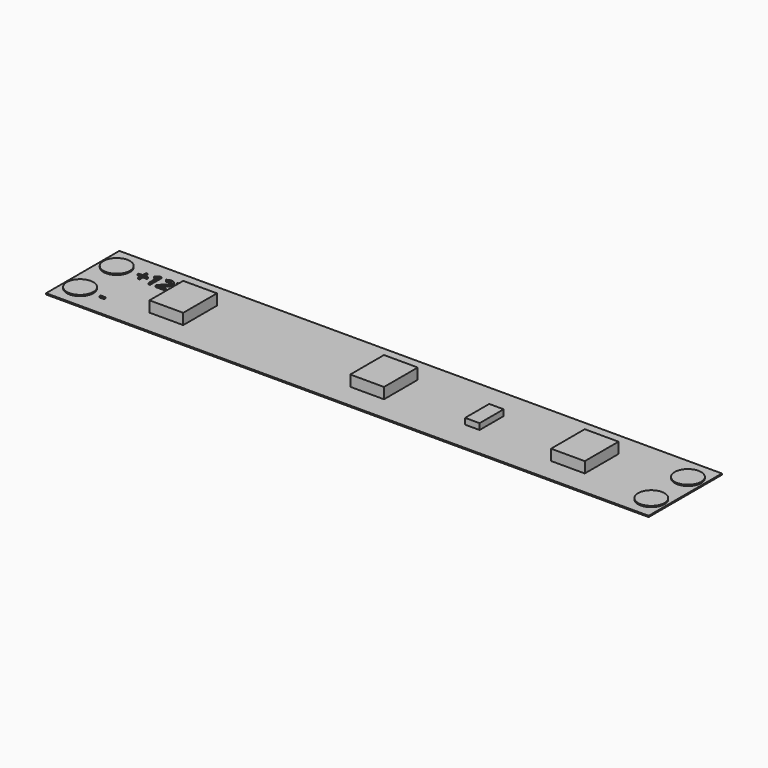
from build123d import *

# Parameters (mm, degrees)
F0_W         = 50
F0_H         = 7.6
F0_R         = 1.1
F0_W_2       = 0.3994791667
F0_H_2       = 0.1236979167
F0_W_3       = 2.8
F0_H_3       = 3.5
F0_W_4       = 1.2
F0_H_4       = 2.5
F0_TEXT_SIZE = 1.6666666667
F1_DEPTH     = 0.1
F2_DEPTH     = 0.9
F3_DEPTH     = 0.9
F4_DEPTH     = 0.5
F5_DEPTH     = 0.1
F6_DEPTH     = 0.1


# Not quite as in the source:
# - Text() gives the source's letters only with a copy of the font that has no kerning and outlines rounded to 1/6400 em; it was checked with that copy


with BuildPart() as f1:
    # F0 (on Top) → F1 (new body)
    with BuildSketch(Plane.XY):
        Rectangle(F0_W, F0_H)
        with Locations((-23.7, -1.9)):
            Circle(F0_R, mode=Mode.SUBTRACT)
        with Locations((-21.7317708333, -2.0532552083)):
            Rectangle(F0_W_2, F0_H_2, mode=Mode.SUBTRACT)
        with Locations((-16.66, 0)):
            Rectangle(F0_W_3, F0_H_3, mode=Mode.SUBTRACT)
        with Locations((23.7, -1.9)):
            Circle(F0_R, mode=Mode.SUBTRACT)
        Rectangle(F0_W_3, F0_H_3, mode=Mode.SUBTRACT)
        with Locations((8.33, 0)):
            Rectangle(F0_W_4, F0_H_4, mode=Mode.SUBTRACT)
        with Locations((16.66, 0)):
            Rectangle(F0_W_3, F0_H_3, mode=Mode.SUBTRACT)
        with Locations((-23.7, 1.9)):
            Circle(F0_R, mode=Mode.SUBTRACT)
        Polygon((-21.4684895833, 2.2919270833), (-21.4684895833, 1.94375), (-21.1333333333, 1.94375), (-21.1333333333, 1.8315104167), (-21.4684895833, 1.8315104167), (-21.4684895833, 1.4846354167), (-21.5817708333, 1.4846354167), (-21.5817708333, 1.8315104167), (-21.9153645833, 1.8315104167), (-21.9153645833, 1.94375), (-21.5817708333, 1.94375), (-21.5817708333, 2.2919270833), align=None, mode=Mode.SUBTRACT)
        with BuildLine():
            Line((-20.4653645833, 2.48984375), (-20.4653645833, 1.3))
            Line((-20.4653645833, 1.3), (-20.5971354167, 1.3))
            Line((-20.5971354167, 1.3), (-20.5971354167, 2.1479166667))
            add(Edge.make_bspline(
                [(-20.5971354167, 2.1479166667), (-20.5971354167, 2.25390625), (-20.590625, 2.3481770833)],
                knots=[0, 0, 0, 1, 1, 1], degree=2))
            add(Edge.make_bspline(
                [(-20.590625, 2.3481770833), (-20.6075520833, 2.3309895833), (-20.6287760417, 2.3123697917)],
                knots=[0, 0, 0, 1, 1, 1], degree=2))
            add(Edge.make_bspline(
                [(-20.6287760417, 2.3123697917), (-20.65, 2.29375), (-20.8223958333, 2.1536458333)],
                knots=[0, 0, 0, 1, 1, 1], degree=2))
            Line((-20.8223958333, 2.1536458333), (-20.8940104167, 2.2463541667))
            Line((-20.8940104167, 2.2463541667), (-20.5791666667, 2.48984375))
            Line((-20.5791666667, 2.48984375), (-20.4653645833, 2.48984375))
        make_face(mode=Mode.SUBTRACT)
        with BuildLine():
            Line((-18.5700520833, 1.7247395833), (-18.2981770833, 2.48984375))
            Line((-18.2981770833, 2.48984375), (-18.1494791667, 2.48984375))
            Line((-18.1494791667, 2.48984375), (-18.578125, 1.3))
            Line((-18.578125, 1.3), (-18.71484375, 1.3))
            Line((-18.71484375, 1.3), (-19.14140625, 2.48984375))
            Line((-19.14140625, 2.48984375), (-18.9947916667, 2.48984375))
            Line((-18.9947916667, 2.48984375), (-18.7213541667, 1.7200520833))
            add(Edge.make_bspline(
                [(-18.7213541667, 1.7200520833), (-18.67421875, 1.5872395833), (-18.6466145833, 1.4619791667)],
                knots=[0, 0, 0, 1, 1, 1], degree=2))
            add(Edge.make_bspline(
                [(-18.6466145833, 1.4619791667), (-18.6171875, 1.59375), (-18.5700520833, 1.7247395833)],
                knots=[0, 0, 0, 1, 1, 1], degree=2))
        make_face(mode=Mode.SUBTRACT)
        with BuildLine():
            Line((-19.2307291667, 1.4252604167), (-19.2307291667, 1.3))
            Line((-19.2307291667, 1.3), (-20.0127604167, 1.3))
            Line((-20.0127604167, 1.3), (-20.0127604167, 1.41640625))
            Line((-20.0127604167, 1.41640625), (-19.6994791667, 1.73125))
            add(Edge.make_bspline(
                [(-19.6994791667, 1.73125), (-19.55625, 1.8763020833), (-19.5106770833, 1.9381510417)],
                knots=[0, 0, 0, 1, 1, 1], degree=2))
            add(Edge.make_bspline(
                [(-19.5106770833, 1.9381510417), (-19.4651041667, 2), (-19.4423177083, 2.05859375)],
                knots=[0, 0, 0, 1, 1, 1], degree=2))
            add(Edge.make_bspline(
                [(-19.4423177083, 2.05859375), (-19.41953125, 2.1171875), (-19.41953125, 2.1846354167)],
                knots=[0, 0, 0, 1, 1, 1], degree=2))
            add(Edge.make_bspline(
                [(-19.41953125, 2.1846354167), (-19.41953125, 2.2799479167), (-19.47734375, 2.3356770833)],
                knots=[0, 0, 0, 1, 1, 1], degree=2))
            add(Edge.make_bspline(
                [(-19.47734375, 2.3356770833), (-19.53515625, 2.39140625), (-19.6377604167, 2.39140625)],
                knots=[0, 0, 0, 1, 1, 1], degree=2))
            add(Edge.make_bspline(
                [(-19.6377604167, 2.39140625), (-19.71171875, 2.39140625), (-19.778125, 2.3669270833)],
                knots=[0, 0, 0, 1, 1, 1], degree=2))
            add(Edge.make_bspline(
                [(-19.778125, 2.3669270833), (-19.84453125, 2.3424479167), (-19.92578125, 2.278125)],
                knots=[0, 0, 0, 1, 1, 1], degree=2))
            Line((-19.92578125, 2.278125), (-19.9973958333, 2.3700520833))
            add(Edge.make_bspline(
                [(-19.9973958333, 2.3700520833), (-19.8330729167, 2.5067708333), (-19.6393229167, 2.5067708333)],
                knots=[0, 0, 0, 1, 1, 1], degree=2))
            add(Edge.make_bspline(
                [(-19.6393229167, 2.5067708333), (-19.4716145833, 2.5067708333), (-19.3764322917, 2.4209635417)],
                knots=[0, 0, 0, 1, 1, 1], degree=2))
            add(Edge.make_bspline(
                [(-19.3764322917, 2.4209635417), (-19.28125, 2.33515625), (-19.28125, 2.1903645833)],
                knots=[0, 0, 0, 1, 1, 1], degree=2))
            add(Edge.make_bspline(
                [(-19.28125, 2.1903645833), (-19.28125, 2.0770833333), (-19.3447916667, 1.96640625)],
                knots=[0, 0, 0, 1, 1, 1], degree=2))
            add(Edge.make_bspline(
                [(-19.3447916667, 1.96640625), (-19.4083333333, 1.8557291667), (-19.5822916667, 1.6864583333)],
                knots=[0, 0, 0, 1, 1, 1], degree=2))
            Line((-19.5822916667, 1.6864583333), (-19.8427083333, 1.4317708333))
            Line((-19.8427083333, 1.4317708333), (-19.8427083333, 1.4252604167))
            Line((-19.8427083333, 1.4252604167), (-19.2307291667, 1.4252604167))
        make_face(mode=Mode.SUBTRACT)
        with Locations((23.7, 1.9)):
            Circle(F0_R, mode=Mode.SUBTRACT)
        with Locations((-23.7, -1.9)):
            Circle(F0_R)
        with Locations((-16.66, 0)):
            Rectangle(F0_W_3, F0_H_3)
        with Locations((-23.7, 1.9)):
            Circle(F0_R)
        Rectangle(F0_W_3, F0_H_3)
        with Locations((8.33, 0)):
            Rectangle(F0_W_4, F0_H_4)
        with Locations((16.66, 0)):
            Rectangle(F0_W_3, F0_H_3)
        with Locations((23.7, -1.9)):
            Circle(F0_R)
        with Locations((23.7, 1.9)):
            Circle(F0_R)
        with Locations((-22, 1.3)):
            Text('+12V', F0_TEXT_SIZE, font='Open Sans', text_align=(TextAlign.LEFT, TextAlign.BOTTOM))
        with Locations((-22, -2.5)):
            Text('-', F0_TEXT_SIZE, font='Open Sans', text_align=(TextAlign.LEFT, TextAlign.BOTTOM))
    extrude(amount=-F1_DEPTH)

    # F0 (on Top) → F6 (join)
    with BuildSketch(Plane.XY):
        with Locations((-22, 1.3)):
            Text('+12V', F0_TEXT_SIZE, font='Open Sans', text_align=(TextAlign.LEFT, TextAlign.BOTTOM))
        with Locations((-22, -2.5)):
            Text('-', F0_TEXT_SIZE, font='Open Sans', text_align=(TextAlign.LEFT, TextAlign.BOTTOM))
    extrude(amount=F6_DEPTH)


with BuildPart() as f2:
    # F0 (on Top) → F2 (new body)
    with BuildSketch(Plane.XY):
        with Locations((-16.66, 0)):
            Rectangle(F0_W_3, F0_H_3)
    extrude(amount=F2_DEPTH)


with BuildPart() as f3:
    # F0 (on Top) → F3 (new body)
    with BuildSketch(Plane.XY):
        Rectangle(F0_W_3, F0_H_3)
    extrude(amount=F3_DEPTH)


with BuildPart() as f3b:
    # F0 (on Top) → F3, piece 2 (new body)
    with BuildSketch(Plane.XY):
        with Locations((16.66, 0)):
            Rectangle(F0_W_3, F0_H_3)
    extrude(amount=F3_DEPTH)


with BuildPart() as f4:
    # F0 (on Top) → F4 (new body)
    with BuildSketch(Plane.XY):
        with Locations((8.33, 0)):
            Rectangle(F0_W_4, F0_H_4)
    extrude(amount=F4_DEPTH)


with BuildPart() as f5:
    # F0 (on Top) → F5 (new body)
    with BuildSketch(Plane.XY):
        with Locations((-23.7, -1.9)):
            Circle(F0_R)
    extrude(amount=F5_DEPTH)


with BuildPart() as f5b:
    # F0 (on Top) → F5, piece 2 (new body)
    with BuildSketch(Plane.XY):
        with Locations((-23.7, 1.9)):
            Circle(F0_R)
    extrude(amount=F5_DEPTH)


with BuildPart() as f5c:
    # F0 (on Top) → F5, piece 3 (new body)
    with BuildSketch(Plane.XY):
        with Locations((23.7, 1.9)):
            Circle(F0_R)
    extrude(amount=F5_DEPTH)


with BuildPart() as f5d:
    # F0 (on Top) → F5, piece 4 (new body)
    with BuildSketch(Plane.XY):
        with Locations((23.7, -1.9)):
            Circle(F0_R)
    extrude(amount=F5_DEPTH)


solid = Compound([f1.part, f2.part, f3.part, f3b.part, f4.part, f5.part, f5b.part, f5c.part, f5d.part])
